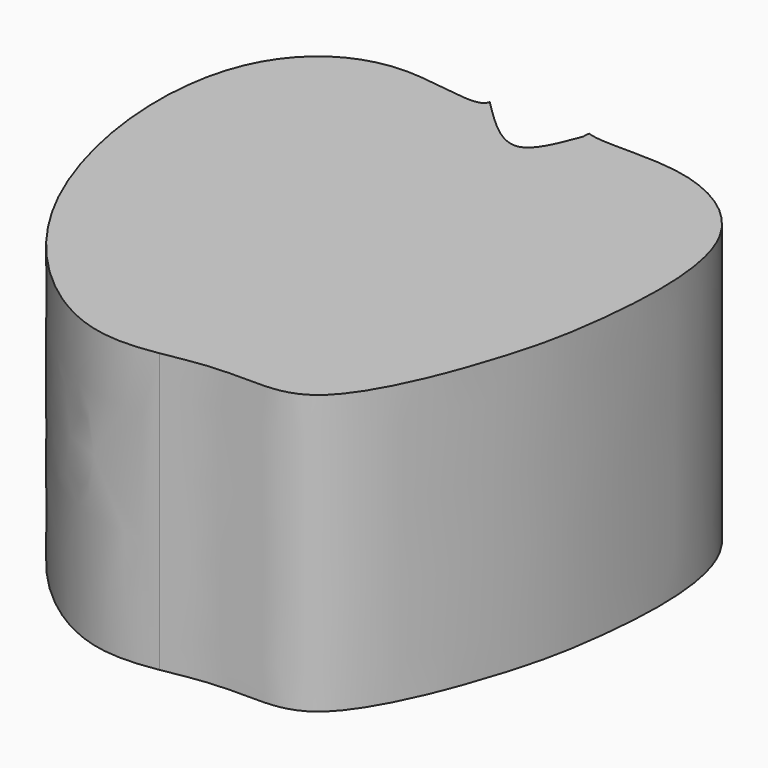
from build123d import *

# Parameters (mm, degrees)
F1_DEPTH = 25.4


with BuildPart() as f1:
    # F0 (on Top) → F1 (new body)
    with BuildSketch(Plane.XY):
        with BuildLine():
            add(Edge.make_bspline(
                [(0, 16.4123084396), (1.2200616504, 16.6464344415), (1.9514227621, 18.5809102283), (2.6827838738, 20.5153860152)],
                knots=[0.5468016302, 0.5468016302, 0.5468016302, 0.5468016302, 1, 1, 1, 1], degree=3))
            Line((0, 16.4123084396), (0, -24.4021035616))
            add(Edge.make_bspline(
                [(2.7344317625, 21.1269656467), (4.3619516884, 20.5278971438), (11.9761249056, 21.7425858169), (22.207718454, 15.2370149441), (21.5670381154, -0.5807645638), (19.6809851156, -9.7595184086), (14.0490357914, -23.8626322199), (7.3445930023, -23.6196180627), (3.5852921603, -23.7099375503), (0.8349352795, -24.2645396907), (0, -24.4021035616)],
                knots=[0.0006542248, 0.0006542248, 0.0006542248, 0.0006542248, 0.0617120582, 0.131283657, 0.2110013704, 0.2798871598, 0.3576074262, 0.4071717299, 0.4546590114, 0.4738187916, 0.4738187916, 0.4738187916, 0.4738187916], degree=3))
            Line((2.7344317625, 21.1269656467), (2.6827838738, 20.9362134337))
            add(Edge.make_bspline(
                [(2.6827838738, 20.9362134337), (2.6827838738, 20.7959376276), (2.6827838738, 20.6556618214), (2.6827838738, 20.5153860152)],
                knots=[0.2104137093, 0.2104137093, 0.2104137093, 0.2104137093, 0.6312411278, 0.6312411278, 0.6312411278, 0.6312411278], degree=3))
        make_face()
        with BuildLine():
            Line((0, -24.4021035616), (0, 16.4123084396))
            add(Edge.make_bspline(
                [(-4.9784243836, 19.6551613061), (-3.0930535372, 17.7882437458), (-1.278294462, 16.1670077439), (0, 16.4123084396)],
                knots=[0.0719723737, 0.0719723737, 0.0719723737, 0.0719723737, 0.5468016302, 0.5468016302, 0.5468016302, 0.5468016302], degree=3))
            add(Edge.make_bspline(
                [(-5.8389957994, 20.5153860152), (-5.5515978909, 20.2267629291), (-5.2641999823, 19.9381398429), (-4.9784243836, 19.6551613061)],
                knots=[0, 0, 0, 0, 0.0719723737, 0.0719723737, 0.0719723737, 0.0719723737], degree=3))
            add(Edge.make_bspline(
                [(0, -24.4021035616), (-1.8515668673, -24.7071675729), (-8.4776442362, -25.3395773837), (-23.1725456339, -11.9704367404), (-26.5380656051, 14.3249040578), (-15.1679246871, 22.4617705994), (-6.143830471, 19.0654599224), (-5.8389957994, 20.5153860152)],
                knots=[0.4738187916, 0.4738187916, 0.4738187916, 0.4738187916, 0.5163078506, 0.60987728, 0.7143042567, 0.7866441933, 0.8459454691, 0.8459454691, 0.8459454691, 0.8459454691], degree=3))
        make_face()
    extrude(amount=F1_DEPTH)


solid = f1.part
